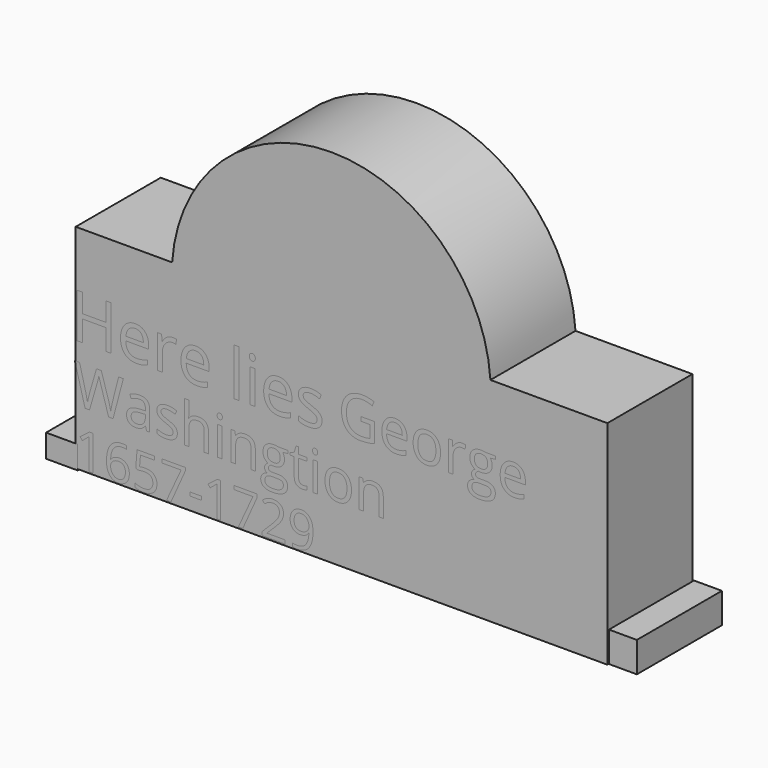
from build123d import *

# Parameters (mm, degrees)
F3_DEPTH       = 25.4
F1_W           = 6.664916873
F1_H           = 7.2433836758
F1_W_2         = 7.5342468917
F1_H_2         = 5.507029593
F2_TEXT_SIZE   = 14.8926965064
F2_TEXT_SIZE_2 = 13.32424193
F2_TEXT_SIZE_3 = 12.8874904476
F2_TEXT_SIZE_4 = 11.7098576286
F4_DEPTH       = 25.4


# Not quite as in the source:
# - Text() gives the source's letters only with a copy of the font that has no kerning and outlines rounded to 1/6400 em; it was checked with that copy


with BuildPart() as f3:
    # F0 (on Front) → F3 (new body)
    with BuildSketch(Plane.XZ):
        Polygon((-39.6453839821, 13.1441370395), (-62.6849516754, 13.1441370395), (-62.6849516754, -37.6558629605), (64.3150483246, -37.6558629605), (64.3150483246, 13.1441370395), (36.3851906836, 13.1441370395), align=None)
        with BuildLine():
            ThreePointArc((36.3851906836, 13.1441370395), (-1.6300966493, 48.7048597804), (-39.6453839821, 13.1441370395))
            Line((-39.6453839821, 13.1441370395), (36.3851906836, 13.1441370395))
        make_face()
    extrude(amount=F3_DEPTH)


with BuildPart() as f3b:
    # F1 (on Front) → F3, piece 2 (new body)
    with BuildSketch(Plane.XZ):
        with Locations((68.0284202099, -33.7698031217)):
            Rectangle(F1_W, F1_H)
    extrude(amount=F3_DEPTH)


with BuildPart() as f3c:
    # F1 (on Front) → F3, piece 3 (new body)
    with BuildSketch(Plane.XZ):
        with Locations((-65.9943390638, -35.1968035102)):
            Rectangle(F1_W_2, F1_H_2)
    extrude(amount=F3_DEPTH)


with BuildPart() as f4:
    # F2 (on Front) → F4 (new body)
    with BuildSketch(Plane.XZ):
        with Locations((-63.8022869825, -10.7227414846)):
            Text('Here lies', F2_TEXT_SIZE, font='Open Sans', text_align=(TextAlign.LEFT, TextAlign.BOTTOM))
        with Locations((0, -9.5934541896)):
            Text('George', F2_TEXT_SIZE_2, font='Open Sans', text_align=(TextAlign.LEFT, TextAlign.BOTTOM))
        with Locations((-63.0604326725, -24.3041925132)):
            Text('Washingtion', F2_TEXT_SIZE_3, font='Open Sans', text_align=(TextAlign.LEFT, TextAlign.BOTTOM))
        with Locations((-62.6927986741, -37.3174846172)):
            Text('1657-1729', F2_TEXT_SIZE_4, font='Open Sans', text_align=(TextAlign.LEFT, TextAlign.BOTTOM))
    extrude(amount=F4_DEPTH)


solid = Compound([f3.part, f3b.part, f3c.part, f4.part])
